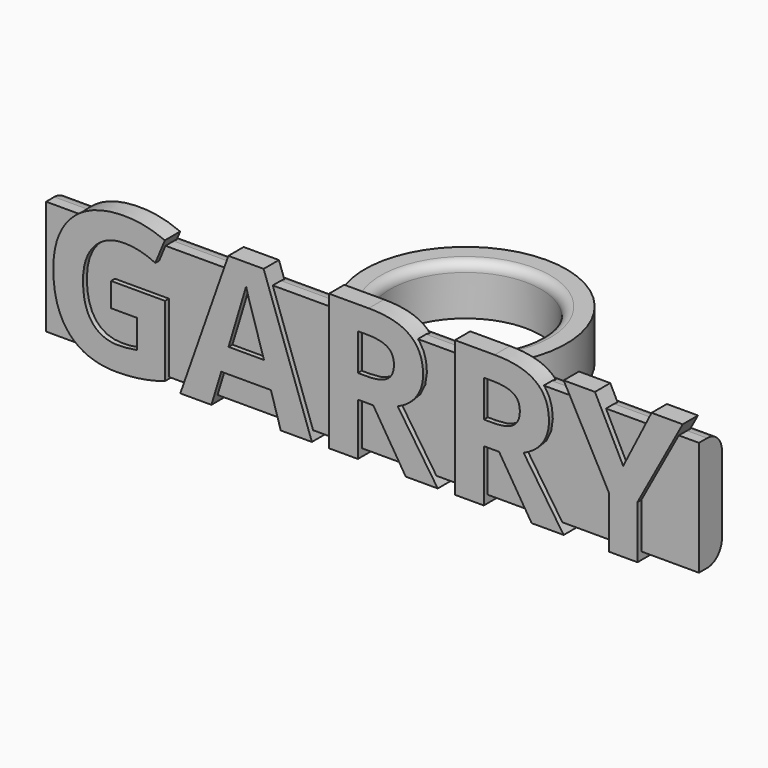
from build123d import *

# Parameters (mm, degrees)
F1_R         = 10.04
F1_R_2       = 7.5
F2_DEPTH     = 2.4765
F4_W         = 2.8629247099
F4_H         = 11.3862990402
F5_DEPTH     = 32.5
F3_TEXT_SIZE = 18.9876306541
F6_DEPTH     = 1.905
F7_R         = 0.9198153673
F8_R         = 1.8396307345


# Not quite as in the source:
# - Text() gives the source's letters only with a copy of the font that has no kerning and outlines rounded to 1/6400 em; it was checked with that copy


with BuildPart() as f2:
    # F1 (on Top) → F2 (new body, symmetric)
    with BuildSketch(Plane.XY):
        Circle(F1_R)
        Circle(F1_R_2, mode=Mode.SUBTRACT)
    extrude(amount=F2_DEPTH, both=True)

    # F4 (on Right) → F5 (join, symmetric)
    with BuildSketch(Plane.YZ):
        with Locations((-10.1516759023, 0.1069603022)):
            Rectangle(F4_W, F4_H)
    extrude(amount=F5_DEPTH, both=True)

    # F7
    f7_edges = [f2.edges().sort_by_distance(p)[0] for p in [
        (-7.5, 0, 2.4765),
    ]]
    fillet(f7_edges, radius=F7_R)

    # F8
    f8_edges = [f2.edges().sort_by_distance(p)[0] for p in [
        (0, -8.720214, -5.586189),
        (0, -8.720214, 5.80011),
    ]]
    fillet(f8_edges, radius=F8_R)


with BuildPart() as f6:
    # F3 (on offset) → F6 (new body)
    with BuildSketch(Plane.XZ.offset(10.16)):
        with Locations((-32.5, -6.3353684287)):
            Text('GARRY', F3_TEXT_SIZE, font='Open Sans', font_style=FontStyle.BOLD, text_align=(TextAlign.LEFT, TextAlign.BOTTOM))
    extrude(amount=F6_DEPTH)


solid = Compound([f2.part, f6.part])
